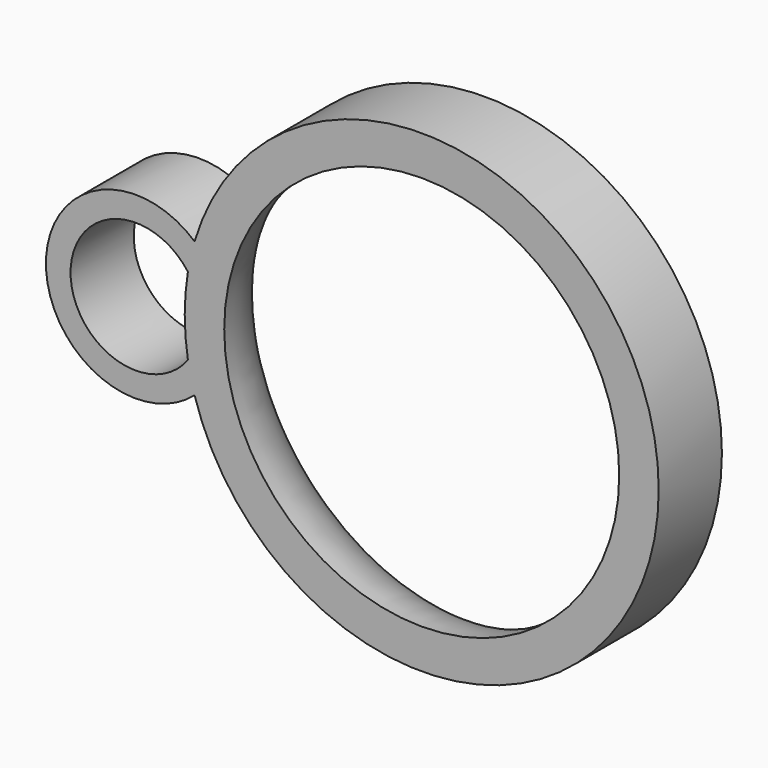
from build123d import *

# Parameters (mm, degrees)
F1_R     = 12
F1_R_2   = 10
F2_DEPTH = 4
F5_DEPTH = 4


# Not quite as in the source:
# - a fillet or chamfer that OpenCascade refuses, or shapes differently, is made with other operations: its cross-section is extruded or revolved along the edge and cut away or added


with BuildPart() as f2:
    # F1 (on Front) → F2 (new body)
    with BuildSketch(Plane.XZ):
        Circle(F1_R)
        Circle(F1_R_2, mode=Mode.SUBTRACT)
    extrude(amount=F2_DEPTH)

    # F3: fillet of radius 5 on 1 edges, made by hand

    # F3_s1 → F3_t2 (revolve, cut)
    with BuildSketch(Plane.XY):
        with BuildLine():
            ThreePointArc((10, -4), (10.527864045, -1.7639320225), (12, 0))
            Line((12, 0), (10, 0))
            Line((10, 0), (10, -4))
        make_face()
    revolve(axis=Axis((0, 0, 0), (0, -1, 0)), mode=Mode.SUBTRACT)

    # F4 (on face) → F5 (join)
    with BuildSketch(Plane.XZ.offset(4)):
        with BuildLine():
            ThreePointArc((-11.8377969718, 1.9663577638), (-11.6917562913, 2.7023757741), (-11.5, 3.4278273002))
            ThreePointArc((-11.5, 3.4278273002), (-19.0279514026, 0), (-11.5, -3.4278273002))
            ThreePointArc((-11.5, -3.4278273002), (-11.6917562913, -2.7023757741), (-11.8377969718, -1.9663577638))
            ThreePointArc((-11.8377969718, -1.9663577638), (-17.78, 0), (-11.8377969718, 1.9663577638))
        make_face()
    extrude(amount=-F5_DEPTH)


solid = f2.part
